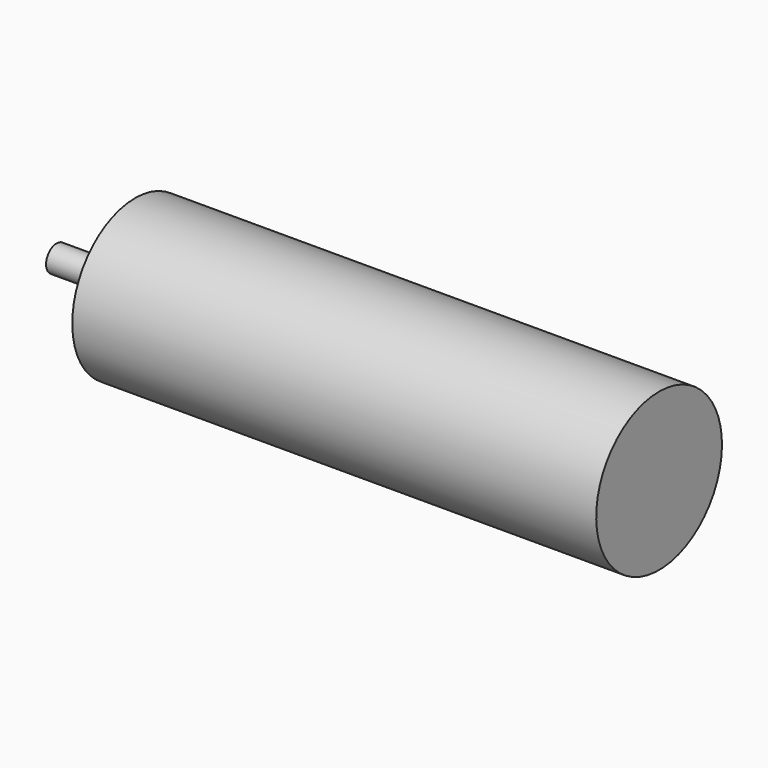
from build123d import *

# Parameters (mm, degrees)
F0_W = 15.24
F0_H = 2.54


# Not quite as in the source:
# - a feature names something its author has since deleted; it is built from what else it names


with BuildPart() as f1:
    # F0 (on Front) → F1 (revolve)
    with BuildSketch(Plane.XZ):
        Polygon((0, 15.24), (-101.6, 15.24), (-101.6, 2.54), (-101.6, 0), (0, 0), align=None)
        with Locations((-109.22, 1.27)):
            Rectangle(F0_W, F0_H)
    revolve(axis=Axis((-50.8, 0, 0), (1, 0, 0)))


solid = f1.part
